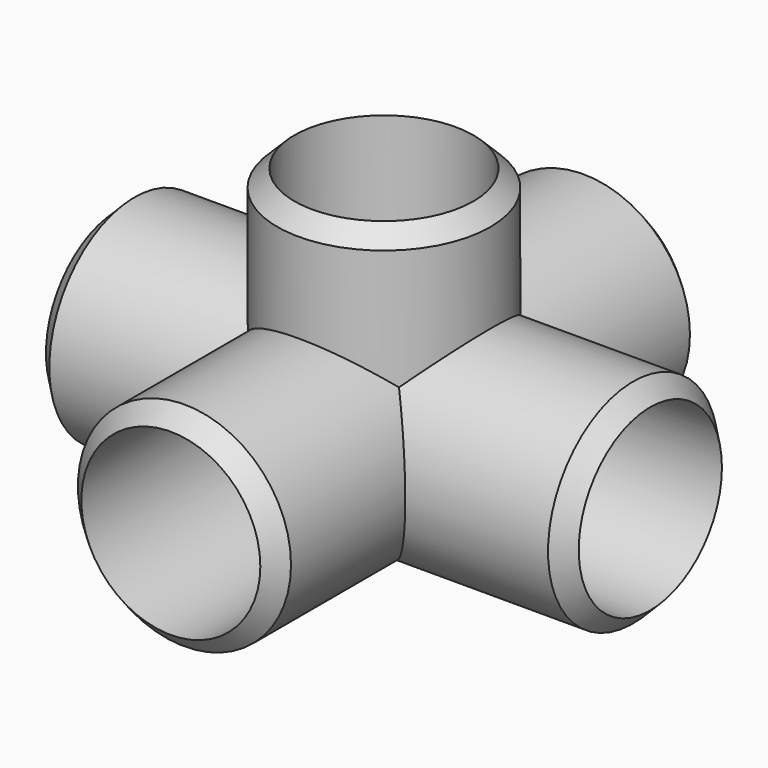
from build123d import *

# Parameters (mm, degrees)
F0_R           = 12.7
F0_R_2         = 10.668
F1_DEPTH       = 31.75
F1_DEPTH_BACK  = 31.75
F2_R           = 12.7
F2_R_2         = 10.668
F3_DEPTH       = 31.75
F3_DEPTH_BACK  = 31.75
F4_R           = 12.7
F4_R_2         = 10.668
F5_DEPTH       = 25.4
F6_SIZE        = 2.03199
F7_R           = 7.8994
F8_DEPTH       = 25.4
F8_DEPTH_BACK  = 25.4
F9_R           = 7.8994
F10_DEPTH      = 25.4
F10_DEPTH_BACK = 25.4
F11_R          = 7.8994
F12_DEPTH      = 25.4


# Not quite as in the source:
# - a fillet or chamfer is up to 0.001 mm smaller than in the source, because OpenCascade refuses the exact size


with BuildPart() as f1:
    # F0 (on Front) → F1 (new body, two sides)
    with BuildSketch(Plane.XZ) as f1_sk:
        Circle(F0_R)
        Circle(F0_R_2, mode=Mode.SUBTRACT)
    extrude(amount=F1_DEPTH)
    extrude(f1_sk.sketch, amount=-F1_DEPTH_BACK)

    # F2 (on Right) → F3 (join, two sides)
    with BuildSketch(Plane.YZ) as f3_sk:
        Circle(F2_R)
        Circle(F2_R_2, mode=Mode.SUBTRACT)
    extrude(amount=F3_DEPTH)
    extrude(f3_sk.sketch, amount=-F3_DEPTH_BACK)

    # F4 (on Top) → F5 (join)
    with BuildSketch(Plane.XY):
        Circle(F4_R)
        Circle(F4_R_2, mode=Mode.SUBTRACT)
    extrude(amount=F5_DEPTH)

    # F6 (size 2.032 in the source; OpenCascade refuses exactly that, so slightly less here)
    f6_edges = [f1.edges().sort_by_distance(p)[0] for p in [
        (-31.75, -12.7, 0),
        (-12.7, -31.75, 0),
        (31.75, -12.7, 0),
        (-12.7, 31.75, 0),
        (-12.7, 0, 25.4),
    ]]
    chamfer(f6_edges, length=F6_SIZE)

    # F7 (on Front) → F8 (cut, two sides)
    with BuildSketch(Plane.XZ) as f8_sk:
        Circle(F7_R)
    extrude(amount=-F8_DEPTH, mode=Mode.SUBTRACT)
    extrude(f8_sk.sketch, amount=F8_DEPTH_BACK, mode=Mode.SUBTRACT)

    # F9 (on Right) → F10 (cut, two sides)
    with BuildSketch(Plane.YZ) as f10_sk:
        Circle(F9_R)
    extrude(amount=-F10_DEPTH, mode=Mode.SUBTRACT)
    extrude(f10_sk.sketch, amount=F10_DEPTH_BACK, mode=Mode.SUBTRACT)

    # F11 (on Top) → F12 (cut)
    with BuildSketch(Plane.XY):
        Circle(F11_R)
    extrude(amount=F12_DEPTH, mode=Mode.SUBTRACT)


solid = f1.part
